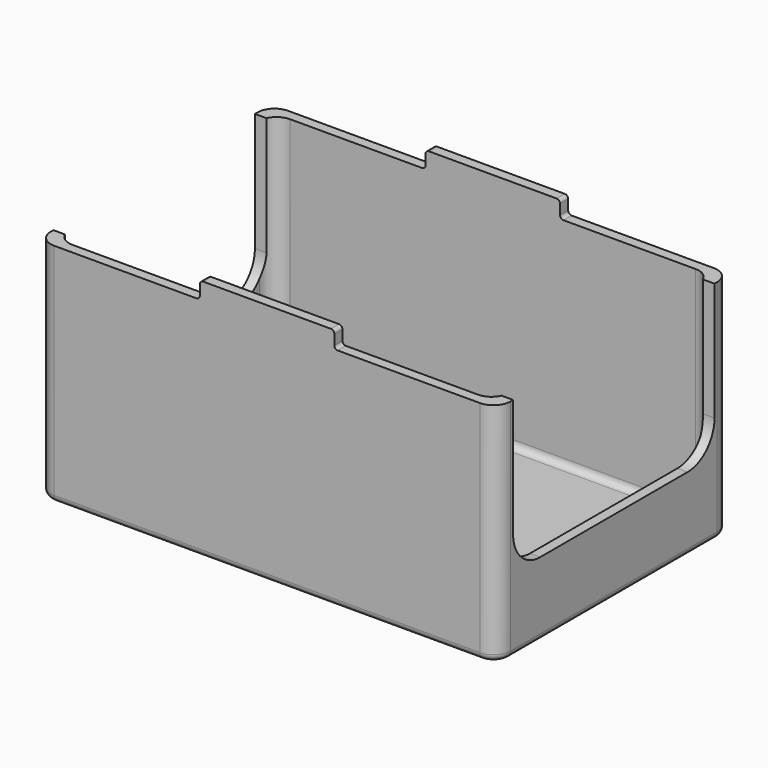
from build123d import *

# Parameters (mm, degrees)
F0_R     = 3
F0_R_2   = 1.4
F0_R_3   = 15
F0_R_4   = 1.5
F1_DEPTH = 3
F0_W     = 65
F0_H     = 3
F2_DEPTH = 67
F4_DEPTH = 136.001
F5_W     = 39.8
F5_H     = 3
F6_W     = 39.8
F6_H     = 3
F7_DEPTH = 5
F8_R     = 1
F9_R     = 5
F10_R    = 2


# Not quite as in the source:
# - a feature names something its author has since deleted; it is built from what else it names


with BuildPart() as f1:
    # F0 (on Top) → F1 (new body)
    with BuildSketch(Plane.XY):
        Polygon((-60.3749420391, 27.6098903269), (-60.3749420391, 7), (-15.3749420391, 7), (-15.3749420391, 12), (24.6250579609, 12), (24.6250579609, 7), (69.6250579609, 7), (69.6250579609, 53.4099719524), (69.6250579609, 87.5), (4.6250579609, 87.5), (-60.3749420391, 87.5), (-60.3749420391, 71.25), align=None)
        with Locations((-30.3749420391, 23.25)):
            Circle(F0_R, mode=Mode.SUBTRACT)
        with Locations((-11.3749420391, 31.25)):
            Circle(F0_R_2, mode=Mode.SUBTRACT)
        with Locations((20.6250579609, 31.25)):
            Circle(F0_R_2, mode=Mode.SUBTRACT)
        with Locations((52.6250579609, 23.25)):
            Circle(F0_R, mode=Mode.SUBTRACT)
        with Locations((-11.3749420391, 63.25)):
            Circle(F0_R_2, mode=Mode.SUBTRACT)
        with BuildLine():
            ThreePointArc((-27.3749420391, 71.25), (-30.3749420391, 68.25), (-33.3749420391, 71.25))
            ThreePointArc((-33.3749420391, 71.25), (-30.3749420391, 74.25), (-27.3749420391, 71.25))
        make_face(mode=Mode.SUBTRACT)
        with Locations((4.6250579609, 47.25)):
            Circle(F0_R_3, mode=Mode.SUBTRACT)
        with Locations((20.6250579609, 63.25)):
            Circle(F0_R_2, mode=Mode.SUBTRACT)
        with Locations((52.6250579609, 71.25)):
            Circle(F0_R, mode=Mode.SUBTRACT)
        Polygon((-15.3749420391, 12), (-15.3749420391, 7), (14.8769766092, 7), (24.6250579609, 7), (24.6250579609, 12), align=None)
        with BuildLine():
            ThreePointArc((-27.3749420391, 71.25), (-30.3749420391, 74.25), (-33.3749420391, 71.25))
            ThreePointArc((-33.3749420391, 71.25), (-30.3749420391, 68.25), (-27.3749420391, 71.25))
        make_face()
        with BuildLine():
            ThreePointArc((-28.8749420391, 71.25), (-30.3749420391, 69.75), (-31.8749420391, 71.25))
            ThreePointArc((-31.8749420391, 71.25), (-30.3749420391, 72.75), (-28.8749420391, 71.25))
        make_face(mode=Mode.SUBTRACT)
        with BuildLine():
            ThreePointArc((-28.8749420391, 71.25), (-30.3749420391, 72.75), (-31.8749420391, 71.25))
            ThreePointArc((-31.8749420391, 71.25), (-30.3749420391, 69.75), (-28.8749420391, 71.25))
        make_face()
        with Locations((52.6250579609, 71.25)):
            Circle(F0_R)
        with Locations((52.6250579609, 71.25)):
            Circle(F0_R_4, mode=Mode.SUBTRACT)
        with Locations((52.6250579609, 71.25)):
            Circle(F0_R_4)
        with Locations((52.6250579609, 23.25)):
            Circle(F0_R)
        with Locations((52.6250579609, 23.25)):
            Circle(F0_R_4, mode=Mode.SUBTRACT)
        with Locations((52.6250579609, 23.25)):
            Circle(F0_R_4)
        with Locations((-30.3749420391, 23.25)):
            Circle(F0_R)
        with Locations((-30.3749420391, 23.25)):
            Circle(F0_R_4, mode=Mode.SUBTRACT)
        with Locations((-30.3749420391, 23.25)):
            Circle(F0_R_4)
    extrude(amount=F1_DEPTH)

    # F0 (on Top) → F2 (join)
    with BuildSketch(Plane.XY):
        Polygon((-63.3749420391, 27.6098903269), (-60.3749420391, 27.6098903269), (-60.3749420391, 71.25), (-60.3749420391, 87.5), (-60.3749420391, 90.5), (-63.3749420391, 90.5), align=None)
        with Locations((-27.8749420391, 89)):
            Rectangle(F0_W, F0_H)
        with Locations((37.1250579609, 89)):
            Rectangle(F0_W, F0_H)
        Polygon((69.6250579609, 87.5), (69.6250579609, 53.4099719524), (72.6250579609, 53.4099719524), (72.6250579609, 90.5), (69.6250579609, 90.5), align=None)
        Polygon((69.6250579609, 7), (69.6250579609, 4), (72.6250579609, 4), (72.6250579609, 53.4099719524), (69.6250579609, 53.4099719524), align=None)
        Polygon((14.8769766092, 4), (69.6250579609, 4), (69.6250579609, 7), (24.6250579609, 7), (14.8769766092, 7), align=None)
        Polygon((-60.3749420391, 7), (-60.3749420391, 4), (14.8769766092, 4), (14.8769766092, 7), (-15.3749420391, 7), align=None)
        Polygon((-63.3749420391, 4), (-60.3749420391, 4), (-60.3749420391, 7), (-60.3749420391, 27.6098903269), (-63.3749420391, 27.6098903269), align=None)
    extrude(amount=F2_DEPTH)

    # F3 (on face) → F4 (cut, through all)
    with BuildSketch(Plane(origin=(-63.3749420391, 0, 0), x_dir=(0, -1, 0), z_dir=(-1, 0, 0))):
        with BuildLine():
            ThreePointArc((-20, 21.9706685841), (-12.9289321881, 24.8996007722), (-10, 31.9706685841))
            ThreePointArc((-10, 31.9706685841), (-20, 41.9706685841), (-30, 31.9706685841))
            ThreePointArc((-30, 31.9706685841), (-27.0710678119, 24.8996007722), (-20, 21.9706685841))
        make_face()
        with BuildLine():
            ThreePointArc((-30, 31.9706685841), (-20, 41.9706685841), (-10, 31.9706685841))
            Line((-10, 31.9706685841), (-10, 67))
            Line((-10, 67), (-30, 67))
            Line((-30, 67), (-30, 31.9706685841))
        make_face()
        with BuildLine():
            ThreePointArc((-74.5, 21.9706685841), (-67.4289321881, 24.8996007722), (-64.5, 31.9706685841))
            ThreePointArc((-64.5, 31.9706685841), (-74.5, 41.9706685841), (-84.5, 31.9706685841))
            ThreePointArc((-84.5, 31.9706685841), (-81.5710678119, 24.8996007722), (-74.5, 21.9706685841))
        make_face()
        with BuildLine():
            Line((-64.5, 31.9706685841), (-30, 31.9706685841))
            Line((-30, 31.9706685841), (-30, 67))
            Line((-30, 67), (-84.5, 67))
            Line((-84.5, 67), (-84.5, 31.9706685841))
            ThreePointArc((-84.5, 31.9706685841), (-74.5, 41.9706685841), (-64.5, 31.9706685841))
        make_face()
        with BuildLine():
            ThreePointArc((-20, 21.9706685841), (-27.0710678119, 24.8996007722), (-30, 31.9706685841))
            Line((-30, 31.9706685841), (-64.5, 31.9706685841))
            ThreePointArc((-64.5, 31.9706685841), (-67.4289321881, 24.8996007722), (-74.5, 21.9706685841))
            Line((-74.5, 21.9706685841), (-20, 21.9706685841))
        make_face()
    extrude(amount=-F4_DEPTH, mode=Mode.SUBTRACT)

    # F5 (on face) + F6 (on face) → F7 (join)
    with BuildSketch(Plane.XY.offset(67)):
        with Locations((4.6250579609, 5.5)):
            Rectangle(F5_W, F5_H)
    with BuildSketch(Plane.XY.offset(67)):
        with Locations((4.6250579609, 89)):
            Rectangle(F6_W, F6_H)
    extrude(amount=F7_DEPTH)

    # F8
    f8_edges = [f1.edges().sort_by_distance(p)[0] for p in [
        (-15.274942, 5.5, 67),
        (-15.274942, 5.5, 72),
        (24.525058, 5.5, 72),
        (24.525058, 5.5, 67),
        (-15.274942, 89, 67),
        (-15.274942, 89, 72),
        (24.525058, 89, 72),
        (24.525058, 89, 67),
    ]]
    fillet(f8_edges, radius=F8_R)

    # F9
    f9_edges = [f1.edges().sort_by_distance(p)[0] for p in [
        (72.625058, 4, 33.5),
        (72.625058, 90.5, 33.5),
        (-63.374942, 90.5, 33.5),
        (-63.374942, 4, 33.5),
        (-60.374942, 7, 35),
        (-60.374942, 87.5, 35),
        (69.625058, 87.5, 35),
        (69.625058, 7, 35),
    ]]
    fillet(f9_edges, radius=F9_R)

    # F10
    f10_edges = [f1.edges().sort_by_distance(p)[0] for p in [
        (4.625058, 87.5, 3),
        (4.625058, 4, 0),
    ]]
    fillet(f10_edges, radius=F10_R)


solid = f1.part
